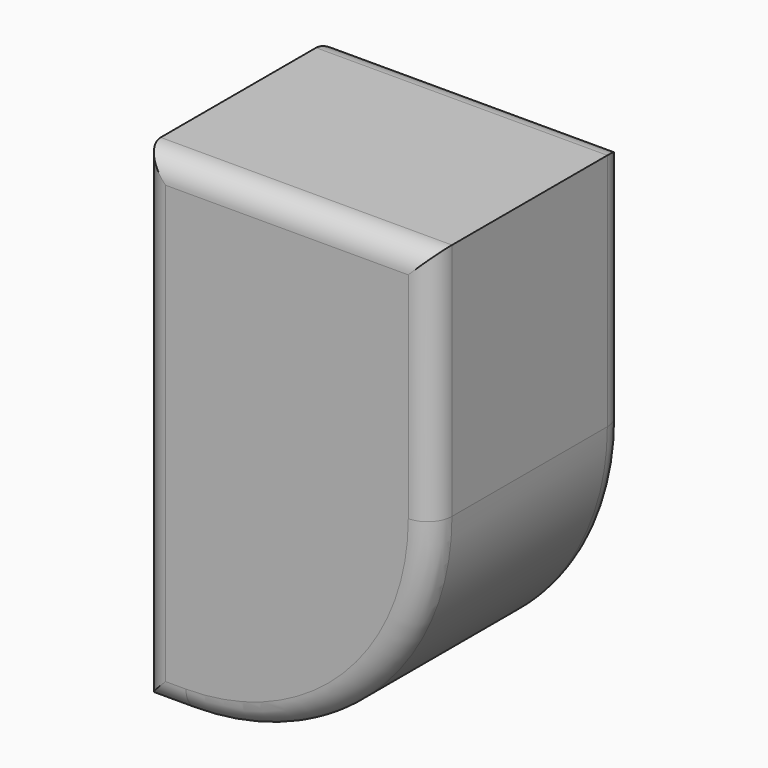
from build123d import *

# Parameters (mm, degrees)
F0_W        = 6
F0_H        = 5
F1_DEPTH    = 10
F2_R        = 0.5
F3_T1_DEPTH = 5
F3_T4_ANGLE = 90
F3_T6_ANGLE = 90


# Not quite as in the source:
# - a fillet or chamfer that OpenCascade refuses, or shapes differently, is made with other operations: its cross-section is extruded or revolved along the edge and cut away or added


with BuildPart() as f1:
    # F0 (on Top) → F1 (new body)
    with BuildSketch(Plane.XY):
        with Locations((3, -2.5)):
            Rectangle(F0_W, F0_H)
    extrude(amount=F1_DEPTH)

    # F2
    f2_edges = [f1.edges().sort_by_distance(p)[0] for p in [
        (6, 0, 5),
        (0, 0, 5),
        (3, 0, 0),
        (3, 0, 10),
        (3, -5, 0),
        (0, -5, 5),
        (6, -5, 5),
        (3, -5, 10),
    ]]
    fillet(f2_edges, radius=F2_R)

    # F3: fillet of radius 5.08 on 1 edges, made by hand

    # F3_s2 → F3_t1 (cut)
    with BuildSketch(Plane.XZ):
        with BuildLine():
            ThreePointArc((6, 5.08), (4.5121024484, 1.4878975516), (0.92, 0))
            Line((0.92, 0), (6, 0))
            Line((6, 0), (6, 5.08))
        make_face()
    extrude(amount=F3_T1_DEPTH, mode=Mode.SUBTRACT)

    # F3_s3 → F3_t4 (revolve, cut)
    with BuildSketch(Plane.YZ.offset(0.92)):
        with BuildLine():
            ThreePointArc((-5, 0.5), (-4.8535533906, 0.1464466094), (-4.5, 0))
            Line((-4.5, 0), (-5, 0))
            Line((-5, 0), (-5, 0.5))
        make_face()
    revolve(axis=Axis((0.92, -5, 5.08), (0, -1, 0)), revolution_arc=F3_T4_ANGLE, mode=Mode.SUBTRACT)

    # F3_s5 → F3_t6 (revolve, cut)
    with BuildSketch(Plane.XY.offset(5.08)):
        with BuildLine():
            ThreePointArc((5.5, 0), (5.8535533906, -0.1464466094), (6, -0.5))
            Line((6, -0.5), (6, 0))
            Line((6, 0), (5.5, 0))
        make_face()
    revolve(axis=Axis((0.92, 0, 5.08), (0, 1, 0)), revolution_arc=F3_T6_ANGLE, mode=Mode.SUBTRACT)


solid = f1.part
